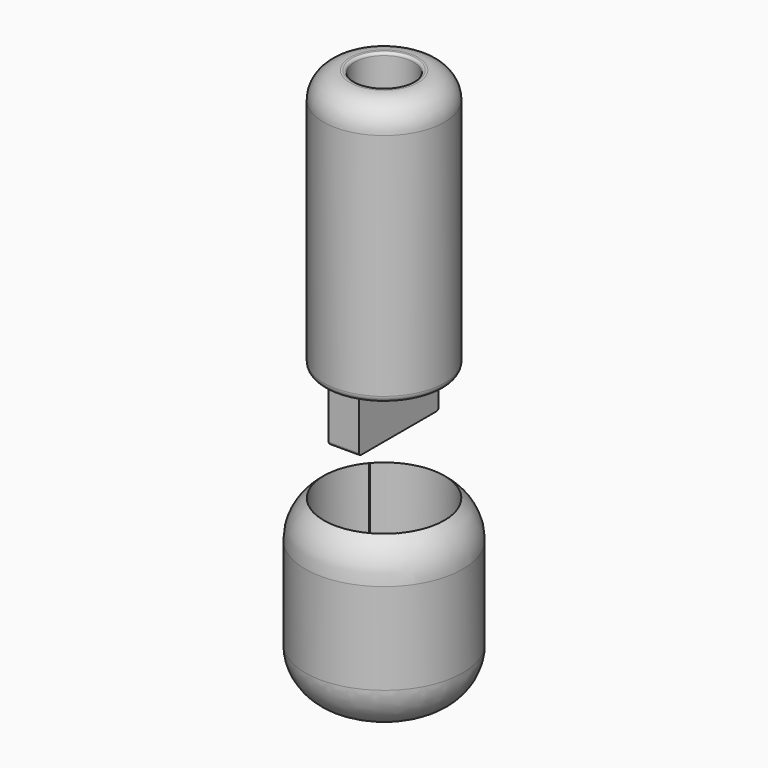
from build123d import *

# Parameters (mm, degrees)
F0_R          = 6
F0_R_2        = 1.75
F1_DEPTH      = 2
F2_DEPTH      = 14
F6_START      = 20
F5_R          = 4.6043307529
F5_R_2        = 2.25
F6_DEPTH      = 20
F7_R          = 2
F8_R          = 0.5
F9_W          = 2.3005146742
F9_H          = 7.5887893885
F10_DEPTH     = 4
F11_T4_ANGLE  = 205.7624022978
F11_T9_ANGLE  = 104.7830244865
F11_T14_ANGLE = 104.7830244865
F12_R         = 0.2


# Not quite as in the source:
# - a fillet or chamfer that OpenCascade refuses, or shapes differently, is made with other operations: its cross-section is extruded or revolved along the edge and cut away or added


with BuildPart() as f1:
    # F0 (on Top) → F1 (new body)
    with BuildSketch(Plane.XY):
        Circle(F0_R)
        with BuildLine():
            Line((-3.4797675825, -3.0085241518), (-3.5099448437, -3.0085241518))
            Line((-3.5099448437, -3.0085241518), (-3.5099448437, -2.973262046))
            ThreePointArc((-3.5099448437, -2.973262046), (-4.6, 0), (-3.5099448437, 2.973262046))
            Line((-3.5099448437, 2.973262046), (-3.5099448437, 3.0085241518))
            Line((-3.5099448437, 3.0085241518), (-3.4797675825, 3.0085241518))
            ThreePointArc((-3.4797675825, 3.0085241518), (0, 4.6), (3.4797675825, 3.0085241518))
            Line((3.4797675825, 3.0085241518), (3.5099448437, 3.0085241518))
            Line((3.5099448437, 3.0085241518), (3.5099448437, 2.973262046))
            ThreePointArc((3.5099448437, 2.973262046), (4.3188972135, 1.583390937), (4.6, 0))
            ThreePointArc((4.6, 0), (4.3188972135, -1.583390937), (3.5099448437, -2.973262046))
            Line((3.5099448437, -2.973262046), (3.5099448437, -3.0085241518))
            Line((3.5099448437, -3.0085241518), (3.4797675825, -3.0085241518))
            ThreePointArc((3.4797675825, -3.0085241518), (0, -4.6), (-3.4797675825, -3.0085241518))
        make_face(mode=Mode.SUBTRACT)
        with BuildLine():
            ThreePointArc((3.4797675825, 3.0085241518), (0, 4.6), (-3.4797675825, 3.0085241518))
            Line((-3.4797675825, 3.0085241518), (3.4797675825, 3.0085241518))
        make_face()
        with BuildLine():
            ThreePointArc((-3.5099448437, 2.973262046), (-4.6, 0), (-3.5099448437, -2.973262046))
            Line((-3.5099448437, -2.973262046), (-3.5099448437, 2.973262046))
        make_face()
        with BuildLine():
            ThreePointArc((-3.5099448437, -2.973262046), (-3.4949006859, -2.9909311586), (-3.4797675825, -3.0085241518))
            Line((-3.4797675825, -3.0085241518), (3.4797675825, -3.0085241518))
            ThreePointArc((3.4797675825, -3.0085241518), (3.4949006859, -2.9909311586), (3.5099448437, -2.973262046))
            Line((3.5099448437, -2.973262046), (3.5099448437, 2.973262046))
            ThreePointArc((3.5099448437, 2.973262046), (3.4949006859, 2.9909311586), (3.4797675825, 3.0085241518))
            Line((3.4797675825, 3.0085241518), (-3.4797675825, 3.0085241518))
            ThreePointArc((-3.4797675825, 3.0085241518), (-3.4949006859, 2.9909311586), (-3.5099448437, 2.973262046))
            Line((-3.5099448437, 2.973262046), (-3.5099448437, -2.973262046))
        make_face()
        Circle(F0_R_2, mode=Mode.SUBTRACT)
        with BuildLine():
            Line((3.4797675825, -3.0085241518), (-3.4797675825, -3.0085241518))
            ThreePointArc((-3.4797675825, -3.0085241518), (0, -4.6), (3.4797675825, -3.0085241518))
        make_face()
        with BuildLine():
            Line((3.5099448437, 2.973262046), (3.5099448437, -2.973262046))
            ThreePointArc((3.5099448437, -2.973262046), (4.3188972135, -1.583390937), (4.6, 0))
            ThreePointArc((4.6, 0), (4.3188972135, 1.583390937), (3.5099448437, 2.973262046))
        make_face()
    extrude(amount=F1_DEPTH)

    # F0 (on Top) → F2 (join)
    with BuildSketch(Plane.XY):
        Circle(F0_R)
        with BuildLine():
            Line((-3.4797675825, -3.0085241518), (-3.5099448437, -3.0085241518))
            Line((-3.5099448437, -3.0085241518), (-3.5099448437, -2.973262046))
            ThreePointArc((-3.5099448437, -2.973262046), (-4.6, 0), (-3.5099448437, 2.973262046))
            Line((-3.5099448437, 2.973262046), (-3.5099448437, 3.0085241518))
            Line((-3.5099448437, 3.0085241518), (-3.4797675825, 3.0085241518))
            ThreePointArc((-3.4797675825, 3.0085241518), (0, 4.6), (3.4797675825, 3.0085241518))
            Line((3.4797675825, 3.0085241518), (3.5099448437, 3.0085241518))
            Line((3.5099448437, 3.0085241518), (3.5099448437, 2.973262046))
            ThreePointArc((3.5099448437, 2.973262046), (4.3188972135, 1.583390937), (4.6, 0))
            ThreePointArc((4.6, 0), (4.3188972135, -1.583390937), (3.5099448437, -2.973262046))
            Line((3.5099448437, -2.973262046), (3.5099448437, -3.0085241518))
            Line((3.5099448437, -3.0085241518), (3.4797675825, -3.0085241518))
            ThreePointArc((3.4797675825, -3.0085241518), (0, -4.6), (-3.4797675825, -3.0085241518))
        make_face(mode=Mode.SUBTRACT)
    extrude(amount=F2_DEPTH)

    # F3: fillet of radius 3.5 on 1 edges, made by hand

    # F3_s1 → F3_t2 (revolve, cut)
    with BuildSketch(Plane.XZ):
        with BuildLine():
            ThreePointArc((6, 3.5), (4.9748737342, 1.0251262658), (2.5, 0))
            Line((2.5, 0), (6, 0))
            Line((6, 0), (6, 3.5))
        make_face()
    revolve(axis=Axis((0, 0, 0), (0, 0, 1)), mode=Mode.SUBTRACT)

    # F4: fillet of radius 3.54 on 1 edges, made by hand

    # F4_s1 → F4_t2 (revolve, cut)
    with BuildSketch(Plane.XZ):
        with BuildLine():
            ThreePointArc((6, 10.46), (4.9631580054, 12.9631580054), (2.46, 14))
            Line((2.46, 14), (6, 14))
            Line((6, 14), (6, 10.46))
        make_face()
    revolve(axis=Axis((0, 0, 14), (0, 0, 1)), mode=Mode.SUBTRACT)


with BuildPart() as f6:
    # F5 (on face) → F6 (new body)
    with BuildSketch(Plane.XY.offset(2).offset(F6_START)):
        Circle(F5_R)
        Circle(F5_R_2, mode=Mode.SUBTRACT)
    extrude(amount=F6_DEPTH)

    # F7
    f7_edges = [f6.edges().sort_by_distance(p)[0] for p in [
        (-4.604331, 0, 42),
    ]]
    fillet(f7_edges, radius=F7_R)

    # F8
    f8_edges = [f6.edges().sort_by_distance(p)[0] for p in [
        (-4.604331, 0, 22),
    ]]
    fillet(f8_edges, radius=F8_R)

    # F9 (on face) → F10 (join)
    with BuildSketch(Plane(origin=(0, 0, 22), x_dir=(1, 0, 0), z_dir=(0, 0, -1))):
        with Locations((-0.0324622379, 0.0056053058)):
            Rectangle(F9_W, F9_H)
    extrude(amount=F10_DEPTH)

    # F11: fillet of radius 0.7 on 3 edges, made by hand


with BuildPart() as f11_tool2:
    # F11_s3 → F11_t4 (revolve)
    with BuildSketch(Plane(origin=(0, 0, 0), x_dir=(0, 0, 1), z_dir=(0.9748343905, -0.2229302831, 0))):
        with BuildLine():
            ThreePointArc((22, -2.95), (22.2050252532, -2.4550252532), (22.7, -2.25))
            Line((22.7, -2.25), (22, -2.25))
            Line((22, -2.25), (22, -2.95))
        make_face()
    revolve(axis=Axis((0, 0, 22), (0, 0, 1)), revolution_arc=F11_T4_ANGLE)

    split(bisect_by=Plane.YZ.offset(-1.182719575), keep=Keep.BOTTOM)


with BuildPart() as f6_1:
    add(f6.part)

    # F11_t1: cut F11_tool2
    add(f11_tool2.part, mode=Mode.SUBTRACT)


with BuildPart() as f11_tool7:
    # F11_s8 → F11_t9 (revolve)
    with BuildSketch(Plane.XZ):
        with BuildLine():
            ThreePointArc((2.95, 22), (2.4550252532, 22.2050252532), (2.25, 22.7))
            Line((2.25, 22.7), (2.25, 22))
            Line((2.25, 22), (2.95, 22))
        make_face()
    revolve(axis=Axis((0, 0, 22), (0, 0, 1)), revolution_arc=F11_T9_ANGLE)

    split(bisect_by=Plane.YZ.offset(1.1177950992), keep=Keep.TOP)


with BuildPart() as f6_2:
    add(f6_1.part)

    # F11_t6: cut F11_tool7
    add(f11_tool7.part, mode=Mode.SUBTRACT)


with BuildPart() as f11_tool12:
    # F11_s13 → F11_t14 (revolve)
    with BuildSketch(Plane(origin=(0, 0, 0), x_dir=(0, 0, 1), z_dir=(-0.9668990293, 0.2551592976, 0))):
        with BuildLine():
            ThreePointArc((22, -2.95), (22.2050252532, -2.4550252532), (22.7, -2.25))
            Line((22.7, -2.25), (22, -2.25))
            Line((22, -2.25), (22, -2.95))
        make_face()
    revolve(axis=Axis((0, 0, 22), (0, 0, 1)), revolution_arc=F11_T14_ANGLE)

    split(bisect_by=Plane.YZ.offset(1.1177950992), keep=Keep.TOP)


with BuildPart() as f6_3:
    add(f6_2.part)

    # F11_t11: cut F11_tool12
    add(f11_tool12.part, mode=Mode.SUBTRACT)

    # F12
    f12_edges = [f6_3.edges().sort_by_distance(p)[0] for p in [
        (-2.25, 0, 42),
        (-0.032462, -3.8, 18),
        (-0.032462, 3.788789, 18),
    ]]
    fillet(f12_edges, radius=F12_R)


solid = Compound([f1.part, f6_3.part])
